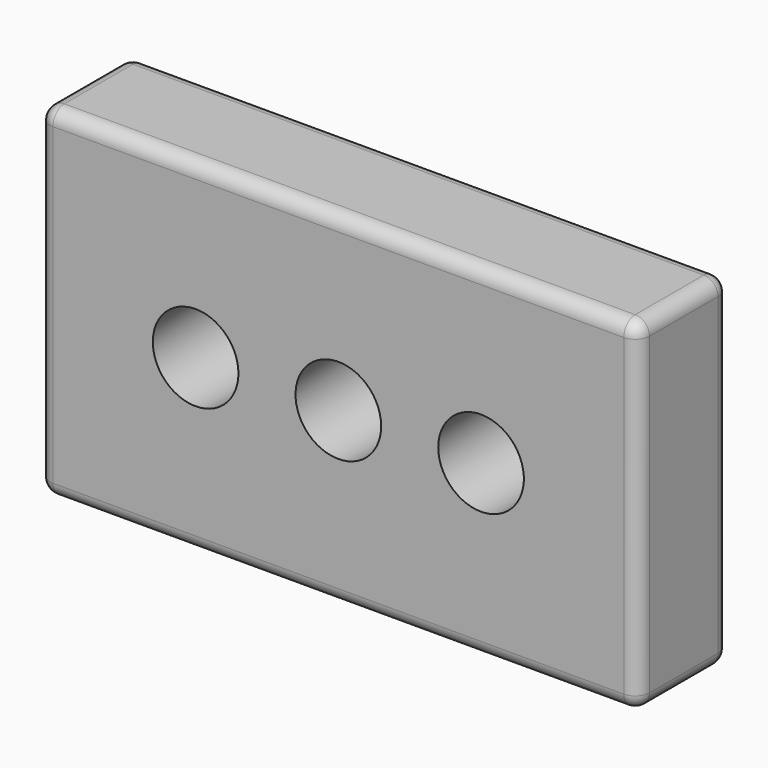
from build123d import *

# Parameters (mm, degrees)
F0_W     = 105
F0_H     = 60
F1_DEPTH = 20
F2_R     = 7.5
F3_DEPTH = 25
F4_R     = 2.5


with BuildPart() as f1:
    # F0 (on Front) → F1 (new body)
    with BuildSketch(Plane.XZ):
        Rectangle(F0_W, F0_H)
    extrude(amount=F1_DEPTH)

    # F2 (on face) → F3 (cut)
    with BuildSketch(Plane.XZ.offset(20)):
        with BuildLine():
            ThreePointArc((-7.5, 0), (0, -7.5), (7.5, 0))
            ThreePointArc((7.5, 0), (0, 7.5), (-7.5, 0))
        make_face()
        with Locations((-25, 0)):
            Circle(F2_R)
        with BuildLine():
            ThreePointArc((32.5, 0), (25, 7.5), (17.5, 0))
            ThreePointArc((17.5, 0), (25, -7.5), (32.5, 0))
        make_face()
    extrude(amount=-F3_DEPTH, mode=Mode.SUBTRACT)

    # F4
    f4_edges = [f1.edges().sort_by_distance(p)[0] for p in [
        (52.5, -10, -30),
        (52.5, -10, 30),
        (52.5, 0, 0),
        (52.5, -20, 0),
        (-52.5, -10, 30),
        (0, 0, 30),
        (0, -20, 30),
        (-52.5, -10, -30),
        (-52.5, 0, 0),
        (-52.5, -20, 0),
        (0, 0, -30),
        (0, -20, -30),
    ]]
    fillet(f4_edges, radius=F4_R)


solid = f1.part
